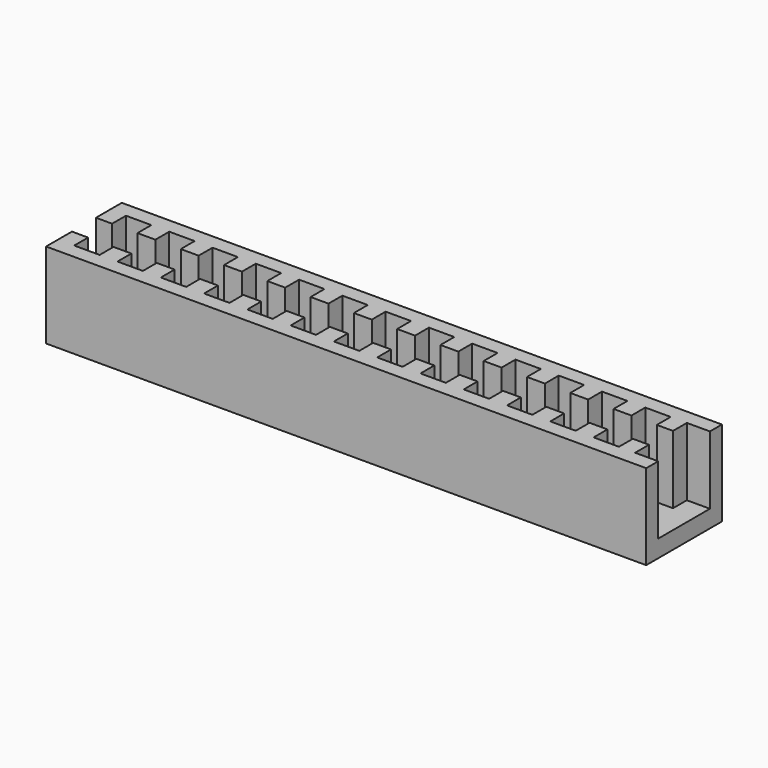
from build123d import *

# Parameters (mm, degrees)
F1_W     = 52
F1_H     = 1.3
F1_H_2   = 5.6
F2_DEPTH = 1.5
F3_DEPTH = 7.4
F4_W     = 1.4
F4_H     = 1.5
F4_W_2   = 0.15
F4_W_3   = 1.25
F5_DEPTH = 5.9


with BuildPart() as f2:
    # F1 (on Top) → F2 (new body)
    with BuildSketch(Plane.XY):
        with Locations((26, -0.65)):
            Rectangle(F1_W, F1_H)
        with Locations((26, -4.1)):
            Rectangle(F1_W, F1_H_2)
        with Locations((26, -7.55)):
            Rectangle(F1_W, F1_H)
    extrude(amount=F2_DEPTH)

    # F1 (on Top) → F3 (join)
    with BuildSketch(Plane.XY):
        with Locations((26, -7.55)):
            Rectangle(F1_W, F1_H)
        with Locations((26, -0.65)):
            Rectangle(F1_W, F1_H)
    extrude(amount=F3_DEPTH)

    # F4 (on face) → F5 (join)
    with BuildSketch(Plane.XY.offset(1.5)):
        with Locations((0.7, -2.05)):
            Rectangle(F4_W, F4_H)
        with Locations((0.7, -6.15)):
            Rectangle(F4_W, F4_H)
        with Locations((3.675, -2.05)):
            Rectangle(F4_W_2, F4_H)
        with Locations((4.375, -2.05)):
            Rectangle(F4_W_3, F4_H)
        with Locations((5.075, -2.05)):
            Rectangle(F4_W_2, F4_H)
        with Locations((3.675, -6.15)):
            Rectangle(F4_W_2, F4_H)
        with Locations((4.375, -6.15)):
            Rectangle(F4_W_3, F4_H)
        with Locations((5.075, -6.15)):
            Rectangle(F4_W_2, F4_H)
        with Locations((7.425, -2.05)):
            Rectangle(F4_W_2, F4_H)
        with Locations((8.125, -2.05)):
            Rectangle(F4_W_3, F4_H)
        with Locations((8.825, -2.05)):
            Rectangle(F4_W_2, F4_H)
        with Locations((7.425, -6.15)):
            Rectangle(F4_W_2, F4_H)
        with Locations((8.125, -6.15)):
            Rectangle(F4_W_3, F4_H)
        with Locations((8.825, -6.15)):
            Rectangle(F4_W_2, F4_H)
        with Locations((11.175, -2.05)):
            Rectangle(F4_W_2, F4_H)
        with Locations((11.875, -2.05)):
            Rectangle(F4_W_3, F4_H)
        with Locations((12.575, -2.05)):
            Rectangle(F4_W_2, F4_H)
        with Locations((11.175, -6.15)):
            Rectangle(F4_W_2, F4_H)
        with Locations((11.875, -6.15)):
            Rectangle(F4_W_3, F4_H)
        with Locations((12.575, -6.15)):
            Rectangle(F4_W_2, F4_H)
        with Locations((14.925, -2.05)):
            Rectangle(F4_W_2, F4_H)
        with Locations((15.625, -2.05)):
            Rectangle(F4_W_3, F4_H)
        with Locations((16.325, -2.05)):
            Rectangle(F4_W_2, F4_H)
        with Locations((14.925, -6.15)):
            Rectangle(F4_W_2, F4_H)
        with Locations((15.625, -6.15)):
            Rectangle(F4_W_3, F4_H)
        with Locations((16.325, -6.15)):
            Rectangle(F4_W_2, F4_H)
        with Locations((18.675, -2.05)):
            Rectangle(F4_W_2, F4_H)
        with Locations((19.375, -2.05)):
            Rectangle(F4_W_3, F4_H)
        with Locations((20.075, -2.05)):
            Rectangle(F4_W_2, F4_H)
        with Locations((18.675, -6.15)):
            Rectangle(F4_W_2, F4_H)
        with Locations((19.375, -6.15)):
            Rectangle(F4_W_3, F4_H)
        with Locations((20.075, -6.15)):
            Rectangle(F4_W_2, F4_H)
        with Locations((22.425, -2.05)):
            Rectangle(F4_W_2, F4_H)
        with Locations((23.125, -2.05)):
            Rectangle(F4_W_3, F4_H)
        with Locations((23.825, -2.05)):
            Rectangle(F4_W_2, F4_H)
        with Locations((22.425, -6.15)):
            Rectangle(F4_W_2, F4_H)
        with Locations((23.125, -6.15)):
            Rectangle(F4_W_3, F4_H)
        with Locations((23.825, -6.15)):
            Rectangle(F4_W_2, F4_H)
        with Locations((26.175, -2.05)):
            Rectangle(F4_W_2, F4_H)
        with Locations((26.875, -2.05)):
            Rectangle(F4_W_3, F4_H)
        with Locations((27.575, -2.05)):
            Rectangle(F4_W_2, F4_H)
        with Locations((26.175, -6.15)):
            Rectangle(F4_W_2, F4_H)
        with Locations((26.875, -6.15)):
            Rectangle(F4_W_3, F4_H)
        with Locations((27.575, -6.15)):
            Rectangle(F4_W_2, F4_H)
        with Locations((29.925, -2.05)):
            Rectangle(F4_W_2, F4_H)
        with Locations((30.625, -2.05)):
            Rectangle(F4_W_3, F4_H)
        with Locations((31.325, -2.05)):
            Rectangle(F4_W_2, F4_H)
        with Locations((29.925, -6.15)):
            Rectangle(F4_W_2, F4_H)
        with Locations((30.625, -6.15)):
            Rectangle(F4_W_3, F4_H)
        with Locations((31.325, -6.15)):
            Rectangle(F4_W_2, F4_H)
        with Locations((33.675, -2.05)):
            Rectangle(F4_W_2, F4_H)
        with Locations((34.375, -2.05)):
            Rectangle(F4_W_3, F4_H)
        with Locations((35.075, -2.05)):
            Rectangle(F4_W_2, F4_H)
        with Locations((33.675, -6.15)):
            Rectangle(F4_W_2, F4_H)
        with Locations((34.375, -6.15)):
            Rectangle(F4_W_3, F4_H)
        with Locations((35.075, -6.15)):
            Rectangle(F4_W_2, F4_H)
        with Locations((37.425, -2.05)):
            Rectangle(F4_W_2, F4_H)
        with Locations((38.125, -2.05)):
            Rectangle(F4_W_3, F4_H)
        with Locations((38.825, -2.05)):
            Rectangle(F4_W_2, F4_H)
        with Locations((37.425, -6.15)):
            Rectangle(F4_W_2, F4_H)
        with Locations((38.125, -6.15)):
            Rectangle(F4_W_3, F4_H)
        with Locations((38.825, -6.15)):
            Rectangle(F4_W_2, F4_H)
        with Locations((41.175, -2.05)):
            Rectangle(F4_W_2, F4_H)
        with Locations((41.875, -2.05)):
            Rectangle(F4_W_3, F4_H)
        with Locations((42.575, -2.05)):
            Rectangle(F4_W_2, F4_H)
        with Locations((41.175, -6.15)):
            Rectangle(F4_W_2, F4_H)
        with Locations((41.875, -6.15)):
            Rectangle(F4_W_3, F4_H)
        with Locations((42.575, -6.15)):
            Rectangle(F4_W_2, F4_H)
        with Locations((44.925, -2.05)):
            Rectangle(F4_W_2, F4_H)
        with Locations((45.625, -2.05)):
            Rectangle(F4_W_3, F4_H)
        with Locations((46.325, -2.05)):
            Rectangle(F4_W_2, F4_H)
        with Locations((44.925, -6.15)):
            Rectangle(F4_W_2, F4_H)
        with Locations((45.625, -6.15)):
            Rectangle(F4_W_3, F4_H)
        with Locations((46.325, -6.15)):
            Rectangle(F4_W_2, F4_H)
        with Locations((49.3, -2.05)):
            Rectangle(F4_W, F4_H)
        with Locations((49.3, -6.15)):
            Rectangle(F4_W, F4_H)
    extrude(amount=F5_DEPTH)


solid = f2.part
